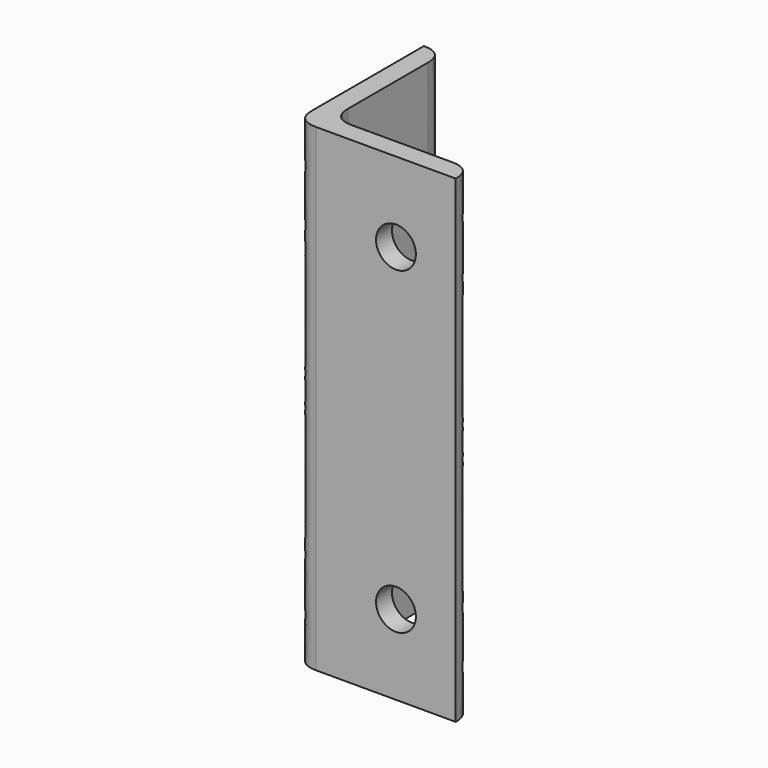
from build123d import *

# Parameters (mm, degrees)
F1_DEPTH    = 76.2
F2_R        = 3.175
F3_DEPTH    = 3.175
F4_T1_DEPTH = 76.2
F4_T3_DEPTH = 92.075


# Not quite as in the source:
# - a fillet or chamfer that OpenCascade refuses, or shapes differently, is made with other operations: its cross-section is extruded or revolved along the edge and cut away or added


with BuildPart() as f1:
    # F0 (on Top) → F1 (new body)
    with BuildSketch(Plane.XY):
        Polygon((-34.0479501394, 7.7857396193), (-37.2229501394, 7.7857396193), (-37.2229501394, -17.6142603807), (-11.8229501394, -17.6142603807), (-11.8229501394, -14.4392603807), (-34.0479501394, -14.4392603807), align=None)
    extrude(amount=F1_DEPTH)

    # F2 (on face) → F3 (cut)
    with BuildSketch(Plane(origin=(0, -14.4392603807, 0), x_dir=(-1, 0, 0), z_dir=(0, 1, 0))):
        with Locations((21.3479501394, 63.5)):
            Circle(F2_R)
        with Locations((21.3479501394, 12.7)):
            Circle(F2_R)
    extrude(amount=-F3_DEPTH, mode=Mode.SUBTRACT)

    # F4: fillet of radius 3.175 on 4 edges, made by hand

    # F4_s2 → F4_t1 (join)
    with BuildSketch(Plane.XY):
        with BuildLine():
            add(Edge.make_bspline(
                [(-34.0479501394, -11.2642603807), (-34.0479501394, -14.4392603807), (-30.8729501394, -14.4392603807)],
                knots=[0, 0, 0, 1, 1, 1], degree=2, weights=[1, 1, 1]))
            Line((-30.8729501394, -14.4392603807), (-34.0479501394, -14.4392603807))
            Line((-34.0479501394, -14.4392603807), (-34.0479501394, -11.2642603807))
        make_face()
    extrude(amount=F4_T1_DEPTH)

    # F4_s4 → F4_t3 (cut)
    with BuildSketch(Plane.XY.offset(-7.9375)):
        with BuildLine():
            add(Edge.make_bspline(
                [(-11.8229501394, -17.6142603807), (-11.8229501394, -14.4392603807), (-14.9979501394, -14.4392603807)],
                knots=[0, 0, 0, 1, 1, 1], degree=2, weights=[1, 1, 1]))
            Line((-14.9979501394, -14.4392603807), (-11.8229501394, -14.4392603807))
            Line((-11.8229501394, -14.4392603807), (-11.8229501394, -17.6142603807))
        make_face()
        with BuildLine():
            add(Edge.make_bspline(
                [(-34.0479501394, 4.6107396193), (-34.0479501394, 7.7857396193), (-37.2229501394, 7.7857396193)],
                knots=[0, 0, 0, 1, 1, 1], degree=2, weights=[1, 1, 1]))
            Line((-37.2229501394, 7.7857396193), (-34.0479501394, 7.7857396193))
            Line((-34.0479501394, 7.7857396193), (-34.0479501394, 4.6107396193))
        make_face()
        with BuildLine():
            add(Edge.make_bspline(
                [(-37.2229501394, -14.4392603807), (-37.2229501394, -17.6142603807), (-34.0479501394, -17.6142603807)],
                knots=[0, 0, 0, 1, 1, 1], degree=2, weights=[1, 1, 1]))
            Line((-34.0479501394, -17.6142603807), (-37.2229501394, -17.6142603807))
            Line((-37.2229501394, -17.6142603807), (-37.2229501394, -14.4392603807))
        make_face()
    extrude(amount=F4_T3_DEPTH, mode=Mode.SUBTRACT)


solid = f1.part
